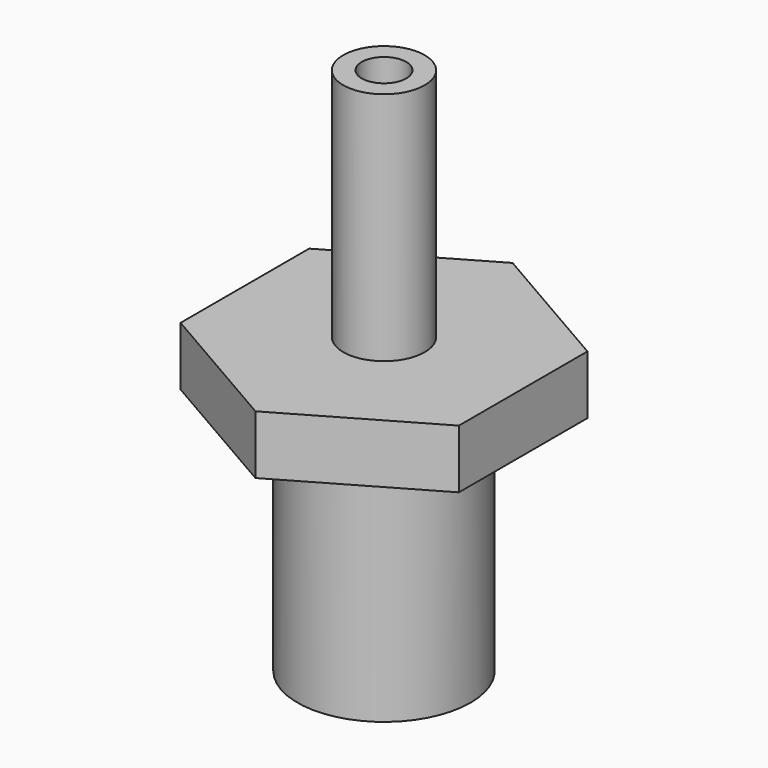
from build123d import *

# Parameters (mm, degrees)
F0_R     = 9.349188324
F0_R_2   = 6.6042884463
F0_R_3   = 4.4026997979
F1_DEPTH = 6.35
F0_R_4   = 2.4090089184
F2_DEPTH = 31.75
F3_DEPTH = 25.4


# Not quite as in the source:
# - a length typed as a fraction of an inch, garbled in the dataset ("3 / 203.2 mm" for 3/8 in), is restored


with BuildPart() as f1:
    # F0 (on Top) → F1 (new body)
    with BuildSketch(Plane.XY):
        Polygon((15.0401592255, -8.6834399775), (15.0401592255, 8.6834399775), (0, 17.366879955), (-15.0401592255, 8.6834399775), (-15.0401592255, -8.6834399775), (0, -17.366879955), align=None)
        Circle(F0_R, mode=Mode.SUBTRACT)
        Circle(F0_R)
        Circle(F0_R_2, mode=Mode.SUBTRACT)
        Circle(F0_R_2)
        Circle(F0_R_3, mode=Mode.SUBTRACT)
    extrude(amount=F1_DEPTH)

    # F0 (on Top) → F2 (join)
    with BuildSketch(Plane.XY):
        Circle(F0_R_3)
        Circle(F0_R_4, mode=Mode.SUBTRACT)
    extrude(amount=F2_DEPTH)

    # F0 (on Top) → F3 (join)
    with BuildSketch(Plane.XY):
        Circle(F0_R)
        Circle(F0_R_2, mode=Mode.SUBTRACT)
    extrude(amount=-F3_DEPTH)


solid = f1.part
